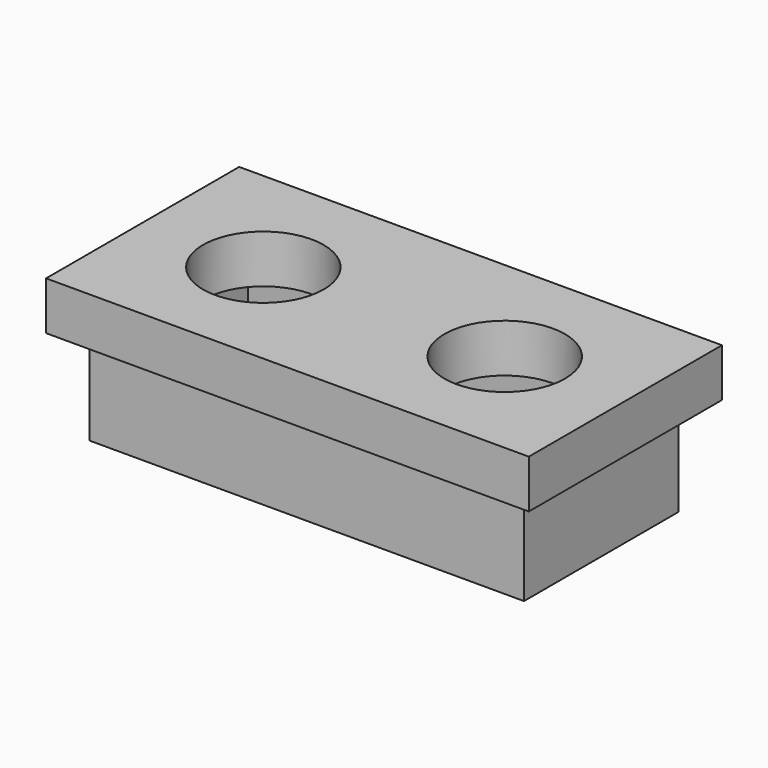
from build123d import *

# Parameters (mm, degrees)
F0_W     = 57.15
F0_H     = 25.4
F1_DEPTH = 12.7
F2_W     = 63.5
F2_H     = 31.75
F2_W_2   = 57.15
F2_H_2   = 25.4
F3_DEPTH = 6.35
F4_R     = 7.9375
F5_DEPTH = 19.051
F6_W     = 52.07
F6_H     = 20.32
F6_R     = 7.9375
F7_DEPTH = 12.7


with BuildPart() as f1:
    # F0 (on Top) → F1 (new body)
    with BuildSketch(Plane.XY):
        Rectangle(F0_W, F0_H)
    extrude(amount=F1_DEPTH)

    # F2 (on face) → F3 (join)
    with BuildSketch(Plane.XY.offset(12.7)):
        Rectangle(F2_W, F2_H)
        Rectangle(F2_W_2, F2_H_2, mode=Mode.SUBTRACT)
        Rectangle(F2_W_2, F2_H_2)
    extrude(amount=F3_DEPTH)

    # F4 (on face) → F5 (cut, through all)
    with BuildSketch(Plane.XY.offset(19.05)):
        with Locations((-15.875, 0)):
            Circle(F4_R)
        with Locations((15.875, 0)):
            Circle(F4_R)
    extrude(amount=-F5_DEPTH, mode=Mode.SUBTRACT)

    # F6 (on face) → F7 (cut)
    with BuildSketch(Plane(origin=(0, 0, 0), x_dir=(1, 0, 0), z_dir=(0, 0, -1))):
        Rectangle(F6_W, F6_H)
        with Locations((-15.875, 0)):
            Circle(F6_R, mode=Mode.SUBTRACT)
        with Locations((15.875, 0)):
            Circle(F6_R, mode=Mode.SUBTRACT)
        with Locations((15.875, 0)):
            Circle(F6_R)
    extrude(amount=-F7_DEPTH, mode=Mode.SUBTRACT)


solid = f1.part
